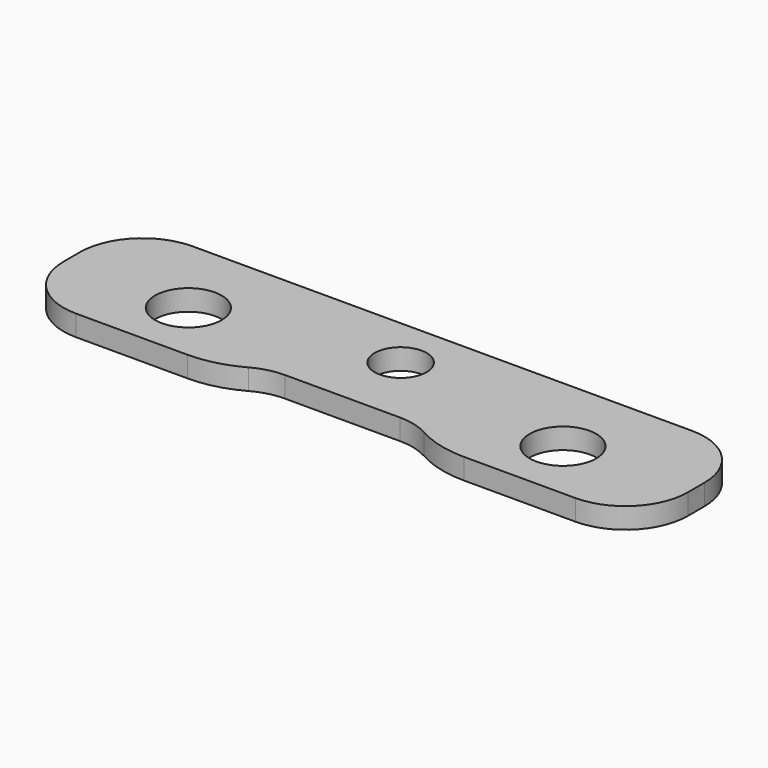
from build123d import *

# Parameters (mm, degrees)
F0_R         = 1.6
F0_R_2       = 1.25
F1_DEPTH     = 1
F2_T1_DEPTH  = 1
F2_T3_DEPTH  = 1
F2_T5_DEPTH  = 16
F2_T7_DEPTH  = 16
F2_T9_DEPTH  = 16
F2_T11_DEPTH = 16
F3_R         = 5


# Not quite as in the source:
# - a fillet or chamfer that OpenCascade refuses, or shapes differently, is made with other operations: its cross-section is extruded or revolved along the edge and cut away or added


with BuildPart() as f1:
    # F0 (on Top) → F1 (new body)
    with BuildSketch(Plane.XY):
        Polygon((15, -3.5), (15, 3.5), (5, 3.5), (-5, 3.5), (-15, 3.5), (-15, -3.5), (-5, -3.5), (-5, -2.5), (5, -2.5), (5, -3.5), align=None)
        with Locations((-9, -0.5)):
            Circle(F0_R, mode=Mode.SUBTRACT)
        with Locations((9, -0.5)):
            Circle(F0_R, mode=Mode.SUBTRACT)
        with Locations((0, 1)):
            Circle(F0_R_2, mode=Mode.SUBTRACT)
    extrude(amount=F1_DEPTH)

    # F2: fillet of radius 3 on 6 edges, made by hand

    # F2_s2 → F2_t1 (join)
    with BuildSketch(Plane.XY):
        with BuildLine():
            ThreePointArc((5, -3.5), (3.9886768939, -2.7613872125), (2.7639320225, -2.5))
            Line((2.7639320225, -2.5), (5, -2.5))
            Line((5, -2.5), (5, -3.5))
        make_face()
    extrude(amount=F2_T1_DEPTH)

    # F2_s4 → F2_t3 (join)
    with BuildSketch(Plane.XY):
        with BuildLine():
            ThreePointArc((-5, -3.5), (-3.9886768939, -2.7613872125), (-2.7639320225, -2.5))
            Line((-2.7639320225, -2.5), (-5, -2.5))
            Line((-5, -2.5), (-5, -3.5))
        make_face()
    extrude(amount=F2_T3_DEPTH)

    # F2_s6 → F2_t5 (cut)
    with BuildSketch(Plane.XY.offset(-7.5)):
        with BuildLine():
            ThreePointArc((15, -0.5), (14.1213203436, -2.6213203436), (12, -3.5))
            Line((12, -3.5), (15, -3.5))
            Line((15, -3.5), (15, -0.5))
        make_face()
    extrude(amount=F2_T5_DEPTH, mode=Mode.SUBTRACT)

    # F2_s8 → F2_t7 (cut)
    with BuildSketch(Plane.XY.offset(-7.5)):
        with BuildLine():
            ThreePointArc((15, 0.5), (14.1213203436, 2.6213203436), (12, 3.5))
            Line((12, 3.5), (15, 3.5))
            Line((15, 3.5), (15, 0.5))
        make_face()
    extrude(amount=F2_T7_DEPTH, mode=Mode.SUBTRACT)

    # F2_s10 → F2_t9 (cut)
    with BuildSketch(Plane.XY.offset(-7.5)):
        with BuildLine():
            ThreePointArc((-12, -3.5), (-14.1213203436, -2.6213203436), (-15, -0.5))
            Line((-15, -0.5), (-15, -3.5))
            Line((-15, -3.5), (-12, -3.5))
        make_face()
    extrude(amount=F2_T9_DEPTH, mode=Mode.SUBTRACT)

    # F2_s12 → F2_t11 (cut)
    with BuildSketch(Plane.XY.offset(-7.5)):
        with BuildLine():
            ThreePointArc((-15, 0.5), (-14.1213203436, 2.6213203436), (-12, 3.5))
            Line((-12, 3.5), (-15, 3.5))
            Line((-15, 3.5), (-15, 0.5))
        make_face()
    extrude(amount=F2_T11_DEPTH, mode=Mode.SUBTRACT)

    # F3
    f3_edges = [f1.edges().sort_by_distance(p)[0] for p in [
        (-5, -3.5, 0.5),
        (5, -3.5, 0.5),
    ]]
    fillet(f3_edges, radius=F3_R)


solid = f1.part
